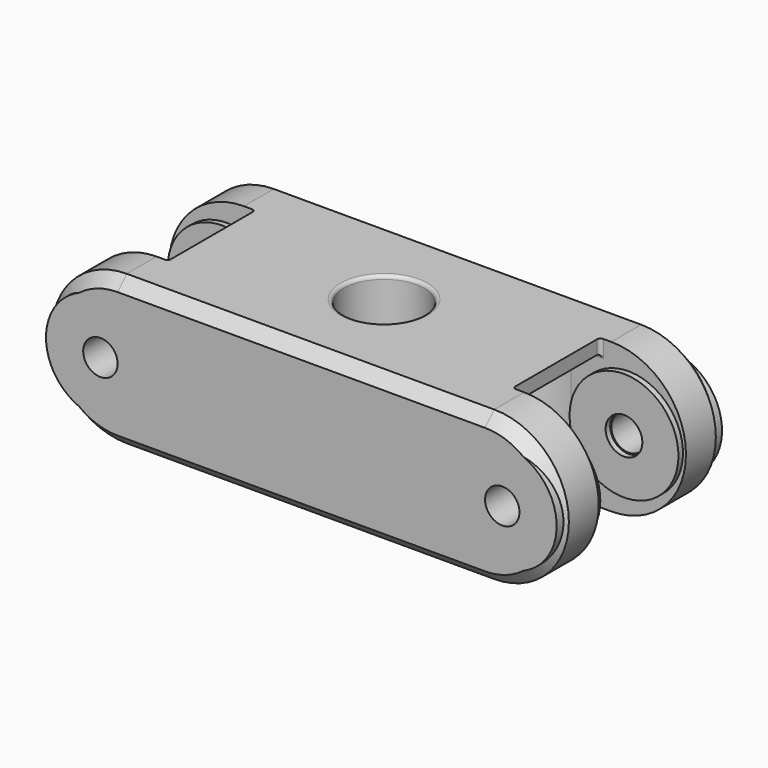
from build123d import *

# Parameters (mm, degrees)
F0_R      = 1.5
F1_DEPTH  = 18
F2_R      = 3.5
F3_DEPTH  = 13.0010005072
F5_DEPTH  = 13.0010005072
F7_DEPTH  = 1.2
F9_DEPTH  = 1.2
F10_R     = 0.3
F11_SIZE  = 1
F12_R     = 4.7403131941
F12_R_2   = 1.6
F13_DEPTH = 4.75
F14_R     = 4.7405
F14_R_2   = 1.6
F15_DEPTH = 4.75


# Not quite as in the source:
# - ends of sketch curves that miss each other by under 0.0002 mm in the source are joined


with BuildPart() as f1:
    # F0 (on Front) → F1 (new body)
    with BuildSketch(Plane.XZ):
        with BuildLine():
            Line((16.0008389681, 6.5000002265), (-16.0008389681, 6.5000002265))
            ThreePointArc((-16.0008389681, 6.5000002265), (-22.5000002671, -0.0004194841), (-16, -6.5000002807))
            Line((-16, -6.5000002807), (16.0016779362, -6.4999997735))
            ThreePointArc((16.0016779362, -6.4999997735), (22.5016782033, 0.0004194841), (16.0008389681, 6.5000002265))
        make_face()
        with Locations((-17.5, 0)):
            Circle(F0_R, mode=Mode.SUBTRACT)
        with Locations((17.5, 0)):
            Circle(F0_R, mode=Mode.SUBTRACT)
    extrude(amount=F1_DEPTH)

    # F2 (on face) → F3 (cut, through all)
    with BuildSketch(Plane.XY.offset(6.5000002265)):
        with Locations((0, -9)):
            Circle(F2_R)
    extrude(amount=-F3_DEPTH, mode=Mode.SUBTRACT)

    # F4 (on face) → F5 (cut, through all)
    with BuildSketch(Plane.XY.offset(6.5000002265)):
        with BuildLine():
            Line((-12.5, -4.25), (-23.5, -4.25))
            Line((-23.5, -4.25), (-23.5, -13.75))
            Line((-23.5, -13.75), (-12.5, -13.75))
            ThreePointArc((-12.5, -13.75), (-7.75, -9), (-12.5, -4.25))
        make_face()
        with BuildLine():
            ThreePointArc((12.5, -4.25), (7.75, -9), (12.5, -13.75))
            Line((12.5, -13.75), (23.5, -13.75))
            Line((23.5, -13.75), (23.5, -4.25))
            Line((23.5, -4.25), (12.5, -4.25))
        make_face()
    extrude(amount=-F5_DEPTH, mode=Mode.SUBTRACT)

    # F6 (on face) → F7 (join)
    with BuildSketch(Plane.XY.offset(6.5000002265)):
        with BuildLine():
            Line((-12.5, -4.25), (-15, -4.25))
            Line((-15, -4.25), (-15, -13.75))
            Line((-15, -13.75), (-12.5, -13.75))
            ThreePointArc((-12.5, -13.75), (-7.75, -9), (-12.5, -4.25))
        make_face()
        with BuildLine():
            ThreePointArc((12.5, -4.25), (7.75, -9), (12.5, -13.75))
            Line((12.5, -13.75), (15, -13.75))
            Line((15, -13.75), (15, -4.25))
            Line((15, -4.25), (12.5, -4.25))
        make_face()
    extrude(amount=-F7_DEPTH)

    # F8 (on face) → F9 (join)
    with BuildSketch(Plane(origin=(0, 0, -6.4999997735), x_dir=(1, 0, 0), z_dir=(0, 0, -1))):
        with BuildLine():
            Line((-12.5, 13.75), (-13.5, 13.75))
            Line((-13.5, 13.75), (-13.5, 4.25))
            Line((-13.5, 4.25), (-12.5, 4.25))
            ThreePointArc((-12.5, 4.25), (-7.75, 9), (-12.5, 13.75))
        make_face()
        with BuildLine():
            ThreePointArc((12.5, 13.75), (7.75, 9), (12.5, 4.25))
            Line((12.5, 4.25), (13.5, 4.25))
            Line((13.5, 4.25), (13.5, 13.75))
            Line((13.5, 13.75), (12.5, 13.75))
        make_face()
    extrude(amount=-F9_DEPTH)

    # F10
    f10_edges = [f1.edges().sort_by_distance(p)[0] for p in [
        (-15, -4.25, 5.9),
        (-13.5, -4.25, -5.9),
        (-13.75, -4.25, 5.3),
        (-15, -13.75, 5.9),
        (-13.5, -13.75, -5.9),
        (-13, -13.75, -5.3),
        (15, -13.75, 5.9),
        (13.75, -13.75, 5.3),
        (13.5, -13.75, -5.9),
        (15, -4.25, 5.9),
        (13.5, -4.25, -5.9),
        (13, -4.25, -5.3),
        (-3.5, -9, 6.5),
        (-3.5, -9, -6.5),
    ]]
    fillet(f10_edges, radius=F10_R)

    # F11
    f11_edges = [f1.edges().sort_by_distance(p)[0] for p in [
        (0, -18, 6.5),
        (0.000839, 0, -6.5),
    ]]
    chamfer(f11_edges, length=F11_SIZE)

    # F12 (on face) → F13 (join)
    with BuildSketch(Plane.XZ.offset(18)):
        with Locations((-17.5, 0)):
            Circle(F12_R)
        with Locations((-17.5, 0)):
            Circle(F12_R_2, mode=Mode.SUBTRACT)
        with Locations((17.5, 0)):
            Circle(F12_R)
        with Locations((17.5, 0)):
            Circle(F12_R_2, mode=Mode.SUBTRACT)
    extrude(amount=-F13_DEPTH)

    # F14 (on face) → F15 (join)
    with BuildSketch(Plane(origin=(0, 0, 0), x_dir=(-1, 0, 0), z_dir=(0, 1, 0))):
        with Locations((17.5, 0)):
            Circle(F14_R)
        with Locations((17.5, 0)):
            Circle(F14_R_2, mode=Mode.SUBTRACT)
        with Locations((-17.5, 0)):
            Circle(F14_R)
        with Locations((-17.5, 0)):
            Circle(F14_R_2, mode=Mode.SUBTRACT)
    extrude(amount=-F15_DEPTH)


solid = f1.part
